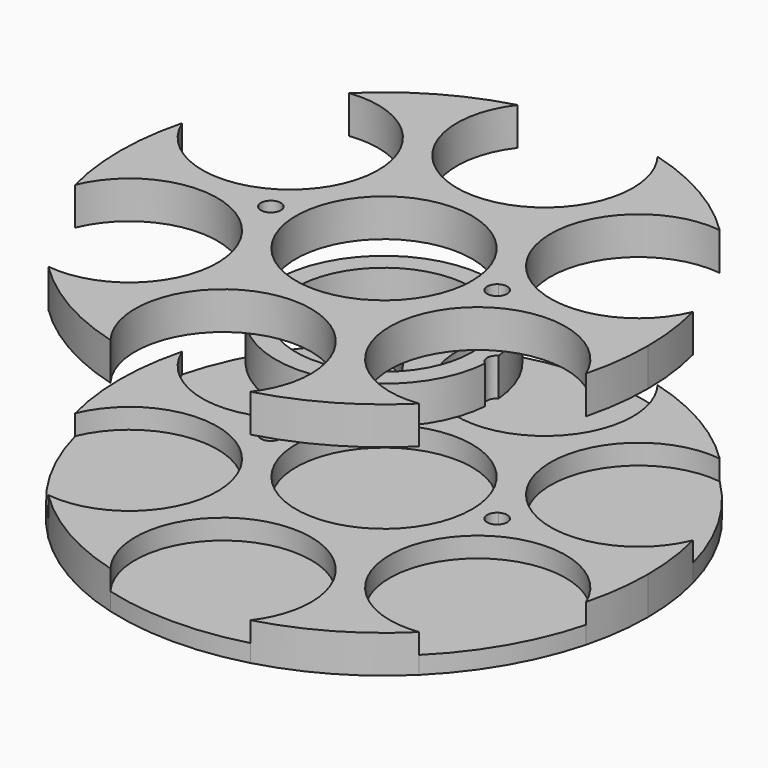
from build123d import *

# Parameters (mm, degrees)
F0_R     = 35
F1_DEPTH = 15
F2_START = -65
F2_DEPTH = 15
F3_DEPTH = 73
F4_START = -10
F4_DEPTH = 15


with BuildPart() as f1:
    # F0 (on Top) → F1 (new body)
    with BuildSketch(Plane.XY):
        with BuildLine():
            ThreePointArc((-27.8107443266, -101.25), (-11.2165937024, -46.8459953291), (35, -80))
            ThreePointArc((35, -80), (33.1540046709, -91.2165937024), (27.8107443266, -101.25))
            ThreePointArc((27.8107443266, -101.25), (52.5, -90.9326673974), (73.7796999699, -74.709811085))
            ThreePointArc((73.7796999699, -74.709811085), (38.9711431703, -22.5), (101.5904442965, -26.540188915))
            ThreePointArc((101.5904442965, -26.540188915), (104.1441228566, -13.3791507367), (105, 0))
            ThreePointArc((105, 0), (104.1441228566, 13.3791507367), (101.5904442965, 26.540188915))
            ThreePointArc((101.5904442965, 26.540188915), (38.9711431703, 22.5), (73.7796999699, 74.709811085))
            ThreePointArc((73.7796999699, 74.709811085), (52.5, 90.9326673974), (27.8107443266, 101.25))
            ThreePointArc((27.8107443266, 101.25), (33.1540046709, 91.2165937024), (35, 80))
            ThreePointArc((35, 80), (-11.2165937024, 46.8459953291), (-27.8107443266, 101.25))
            ThreePointArc((-27.8107443266, 101.25), (-52.5, 90.9326673974), (-73.7796999699, 74.709811085))
            ThreePointArc((-73.7796999699, 74.709811085), (-46.1781188718, 66.2908574256), (-34.2820323028, 40))
            ThreePointArc((-34.2820323028, 40), (-62.4188850575, 5.6794928667), (-101.5904442965, 26.540188915))
            ThreePointArc((-101.5904442965, 26.540188915), (-105, 0), (-101.5904442965, -26.540188915))
            ThreePointArc((-101.5904442965, -26.540188915), (-62.4188850575, -5.6794928667), (-34.2820323028, -40))
            ThreePointArc((-34.2820323028, -40), (-46.1781188718, -66.2908574256), (-73.7796999699, -74.709811085))
            ThreePointArc((-73.7796999699, -74.709811085), (-52.5, -90.9326673974), (-27.8107443266, -101.25))
        make_face()
        with BuildLine():
            ThreePointArc((-42.8991397367, -3.403878105), (-49, 0), (-42.8991397367, 3.403878105))
            ThreePointArc((-42.8991397367, 3.403878105), (0, 43.0339700272), (42.8991397367, 3.403878105))
            ThreePointArc((42.8991397367, 3.403878105), (46.9489175132, 3.4930961233), (49, 0))
            ThreePointArc((49, 0), (46.9489175132, -3.4930961233), (42.8991397367, -3.403878105))
            ThreePointArc((42.8991397367, -3.403878105), (0, -43.0339700272), (-42.8991397367, -3.403878105))
        make_face(mode=Mode.SUBTRACT)
        with BuildLine():
            ThreePointArc((-42.8991397367, 3.403878105), (-41.5069038767, 1.9489175132), (-41, 0))
            ThreePointArc((-41, 0), (-41.5069038767, -1.9489175132), (-42.8991397367, -3.403878105))
            ThreePointArc((-42.8991397367, -3.403878105), (0, -43.0339700272), (42.8991397367, -3.403878105))
            ThreePointArc((42.8991397367, -3.403878105), (41, 0), (42.8991397367, 3.403878105))
            ThreePointArc((42.8991397367, 3.403878105), (0, 43.0339700272), (-42.8991397367, 3.403878105))
        make_face()
        Circle(F0_R, mode=Mode.SUBTRACT)
    extrude(amount=F1_DEPTH)


with BuildPart() as f2:
    # F0 (on Top) → F2 (new body)
    with BuildSketch(Plane.XY.offset(F2_START)):
        with BuildLine():
            ThreePointArc((27.8107443266, -101.25), (33.1540046709, -91.2165937024), (35, -80))
            ThreePointArc((35, -80), (-11.2165937024, -46.8459953291), (-27.8107443266, -101.25))
            ThreePointArc((-27.8107443266, -101.25), (0, -105), (27.8107443266, -101.25))
        make_face()
        with BuildLine():
            ThreePointArc((-27.8107443266, -101.25), (-11.2165937024, -46.8459953291), (35, -80))
            ThreePointArc((35, -80), (33.1540046709, -91.2165937024), (27.8107443266, -101.25))
            ThreePointArc((27.8107443266, -101.25), (52.5, -90.9326673974), (73.7796999699, -74.709811085))
            ThreePointArc((73.7796999699, -74.709811085), (38.9711431703, -22.5), (101.5904442965, -26.540188915))
            ThreePointArc((101.5904442965, -26.540188915), (104.1441228566, -13.3791507367), (105, 0))
            ThreePointArc((105, 0), (104.1441228566, 13.3791507367), (101.5904442965, 26.540188915))
            ThreePointArc((101.5904442965, 26.540188915), (38.9711431703, 22.5), (73.7796999699, 74.709811085))
            ThreePointArc((73.7796999699, 74.709811085), (52.5, 90.9326673974), (27.8107443266, 101.25))
            ThreePointArc((27.8107443266, 101.25), (33.1540046709, 91.2165937024), (35, 80))
            ThreePointArc((35, 80), (-11.2165937024, 46.8459953291), (-27.8107443266, 101.25))
            ThreePointArc((-27.8107443266, 101.25), (-52.5, 90.9326673974), (-73.7796999699, 74.709811085))
            ThreePointArc((-73.7796999699, 74.709811085), (-46.1781188718, 66.2908574256), (-34.2820323028, 40))
            ThreePointArc((-34.2820323028, 40), (-62.4188850575, 5.6794928667), (-101.5904442965, 26.540188915))
            ThreePointArc((-101.5904442965, 26.540188915), (-105, 0), (-101.5904442965, -26.540188915))
            ThreePointArc((-101.5904442965, -26.540188915), (-62.4188850575, -5.6794928667), (-34.2820323028, -40))
            ThreePointArc((-34.2820323028, -40), (-46.1781188718, -66.2908574256), (-73.7796999699, -74.709811085))
            ThreePointArc((-73.7796999699, -74.709811085), (-52.5, -90.9326673974), (-27.8107443266, -101.25))
        make_face()
        with BuildLine():
            ThreePointArc((-42.8991397367, -3.403878105), (-49, 0), (-42.8991397367, 3.403878105))
            ThreePointArc((-42.8991397367, 3.403878105), (0, 43.0339700272), (42.8991397367, 3.403878105))
            ThreePointArc((42.8991397367, 3.403878105), (46.9489175132, 3.4930961233), (49, 0))
            ThreePointArc((49, 0), (46.9489175132, -3.4930961233), (42.8991397367, -3.403878105))
            ThreePointArc((42.8991397367, -3.403878105), (0, -43.0339700272), (-42.8991397367, -3.403878105))
        make_face(mode=Mode.SUBTRACT)
        with BuildLine():
            ThreePointArc((-101.5904442965, -26.540188915), (-90.9326673974, -52.5), (-73.7796999699, -74.709811085))
            ThreePointArc((-73.7796999699, -74.709811085), (-46.1781188718, -66.2908574256), (-34.2820323028, -40))
            ThreePointArc((-34.2820323028, -40), (-62.4188850575, -5.6794928667), (-101.5904442965, -26.540188915))
        make_face()
        with BuildLine():
            ThreePointArc((101.5904442965, -26.540188915), (38.9711431703, -22.5), (73.7796999699, -74.709811085))
            ThreePointArc((73.7796999699, -74.709811085), (90.9326673974, -52.5), (101.5904442965, -26.540188915))
        make_face()
        with BuildLine():
            ThreePointArc((-73.7796999699, 74.709811085), (-90.9326673974, 52.5), (-101.5904442965, 26.540188915))
            ThreePointArc((-101.5904442965, 26.540188915), (-62.4188850575, 5.6794928667), (-34.2820323028, 40))
            ThreePointArc((-34.2820323028, 40), (-46.1781188718, 66.2908574256), (-73.7796999699, 74.709811085))
        make_face()
        with BuildLine():
            ThreePointArc((73.7796999699, 74.709811085), (38.9711431703, 22.5), (101.5904442965, 26.540188915))
            ThreePointArc((101.5904442965, 26.540188915), (90.9326673974, 52.5), (73.7796999699, 74.709811085))
        make_face()
        with BuildLine():
            ThreePointArc((27.8107443266, 101.25), (0, 105), (-27.8107443266, 101.25))
            ThreePointArc((-27.8107443266, 101.25), (-11.2165937024, 46.8459953291), (35, 80))
            ThreePointArc((35, 80), (33.1540046709, 91.2165937024), (27.8107443266, 101.25))
        make_face()
        with BuildLine():
            ThreePointArc((-42.8991397367, 3.403878105), (-41.5069038767, 1.9489175132), (-41, 0))
            ThreePointArc((-41, 0), (-41.5069038767, -1.9489175132), (-42.8991397367, -3.403878105))
            ThreePointArc((-42.8991397367, -3.403878105), (0, -43.0339700272), (42.8991397367, -3.403878105))
            ThreePointArc((42.8991397367, -3.403878105), (41, 0), (42.8991397367, 3.403878105))
            ThreePointArc((42.8991397367, 3.403878105), (0, 43.0339700272), (-42.8991397367, 3.403878105))
        make_face()
        Circle(F0_R, mode=Mode.SUBTRACT)
        Circle(F0_R)
    extrude(amount=-F2_DEPTH)

    # F0 (on Top) → F3 (cut)
    with BuildSketch(Plane.XY):
        with BuildLine():
            ThreePointArc((-101.5904442965, -26.540188915), (-90.9326673974, -52.5), (-73.7796999699, -74.709811085))
            ThreePointArc((-73.7796999699, -74.709811085), (-46.1781188718, -66.2908574256), (-34.2820323028, -40))
            ThreePointArc((-34.2820323028, -40), (-62.4188850575, -5.6794928667), (-101.5904442965, -26.540188915))
        make_face()
        with BuildLine():
            ThreePointArc((-73.7796999699, 74.709811085), (-90.9326673974, 52.5), (-101.5904442965, 26.540188915))
            ThreePointArc((-101.5904442965, 26.540188915), (-62.4188850575, 5.6794928667), (-34.2820323028, 40))
            ThreePointArc((-34.2820323028, 40), (-46.1781188718, 66.2908574256), (-73.7796999699, 74.709811085))
        make_face()
        with BuildLine():
            ThreePointArc((27.8107443266, 101.25), (0, 105), (-27.8107443266, 101.25))
            ThreePointArc((-27.8107443266, 101.25), (-11.2165937024, 46.8459953291), (35, 80))
            ThreePointArc((35, 80), (33.1540046709, 91.2165937024), (27.8107443266, 101.25))
        make_face()
        with BuildLine():
            ThreePointArc((73.7796999699, 74.709811085), (38.9711431703, 22.5), (101.5904442965, 26.540188915))
            ThreePointArc((101.5904442965, 26.540188915), (90.9326673974, 52.5), (73.7796999699, 74.709811085))
        make_face()
        with BuildLine():
            ThreePointArc((27.8107443266, -101.25), (33.1540046709, -91.2165937024), (35, -80))
            ThreePointArc((35, -80), (-11.2165937024, -46.8459953291), (-27.8107443266, -101.25))
            ThreePointArc((-27.8107443266, -101.25), (0, -105), (27.8107443266, -101.25))
        make_face()
        with BuildLine():
            ThreePointArc((101.5904442965, -26.540188915), (38.9711431703, -22.5), (73.7796999699, -74.709811085))
            ThreePointArc((73.7796999699, -74.709811085), (90.9326673974, -52.5), (101.5904442965, -26.540188915))
        make_face()
        Circle(F0_R)
    extrude(amount=-F3_DEPTH, mode=Mode.SUBTRACT)


with BuildPart() as f4:
    # F0 (on Top) → F4 (new body)
    with BuildSketch(Plane.XY.offset(F4_START)):
        with BuildLine():
            ThreePointArc((-42.8991397367, 3.403878105), (-41.5069038767, 1.9489175132), (-41, 0))
            ThreePointArc((-41, 0), (-41.5069038767, -1.9489175132), (-42.8991397367, -3.403878105))
            ThreePointArc((-42.8991397367, -3.403878105), (0, -43.0339700272), (42.8991397367, -3.403878105))
            ThreePointArc((42.8991397367, -3.403878105), (41, 0), (42.8991397367, 3.403878105))
            ThreePointArc((42.8991397367, 3.403878105), (0, 43.0339700272), (-42.8991397367, 3.403878105))
        make_face()
        Circle(F0_R, mode=Mode.SUBTRACT)
    extrude(amount=-F4_DEPTH)


solid = Compound([f1.part, f2.part, f4.part])
